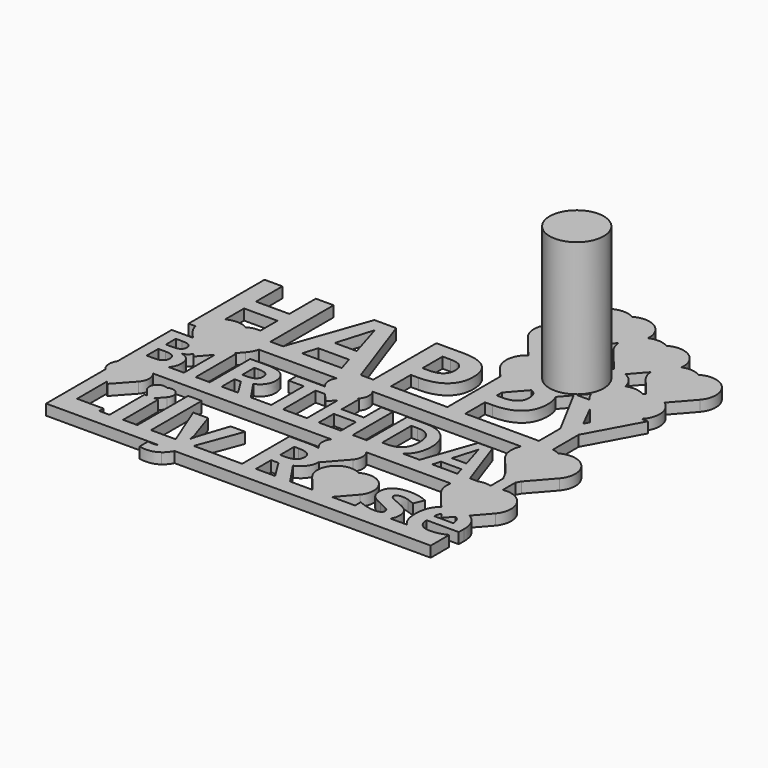
from build123d import *

# Parameters (mm, degrees)
F0_TEXT_SIZE   = 22.0588235294
F0_TEXT_SIZE_2 = 14.6296860713
F0_W           = 2.5421468203
F0_H           = 9.3203158344
F0_H_2         = 12.9721510883
F1_DEPTH       = 2
F2_W           = 69.2715635477
F2_H           = 3
F2_W_2         = 71.8336534358
F2_W_3         = 66.3625919118
F3_DEPTH       = 2
F5_DEPTH       = 2
F6_R           = 5.0531833036
F7_DEPTH       = 25


# Not quite as in the source:
# - Text() gives the source's letters only with a copy of the font that has no kerning and outlines rounded to 1/6400 em; it was checked with that copy


with BuildPart() as f1:
    # F0 (on Top) → F1 (new body)
    with BuildSketch(Plane.XY):
        with Locations((-37.5, 11.5387746485)):
            Text('HAPPY', F0_TEXT_SIZE, font='Open Sans', font_style=FontStyle.BOLD, text_align=(TextAlign.LEFT, TextAlign.BOTTOM))
        with Locations((-37.5, -3.9945993228)):
            Text('BIRTHDAY', F0_TEXT_SIZE_2, font='Open Sans', font_style=FontStyle.BOLD, text_align=(TextAlign.LEFT, TextAlign.BOTTOM))
        Polygon((-35.9661758429, -9.0986326135), (-35.9661758429, -21.2865327415), (-28.4384336321, -21.2865327415), (-28.4384336321, -19.152516523), (-33.3813486983, -19.152516523), (-33.3813486983, -9.0986326135), align=None)
        with Locations((-25.2494131455, -16.6263748243)):
            Rectangle(F0_W, F0_H)
        with Locations((-20.0397460521, -14.8004571973)):
            Rectangle(F0_W, F0_H_2)
        with BuildLine():
            Line((-14.6500213402, -11.9662169071), (-17.4349125053, -11.9662169071))
            Line((-17.4349125053, -11.9662169071), (-13.7323943662, -21.2198447347))
            Line((-13.7323943662, -21.2198447347), (-13.8844430218, -21.6786582217))
            add(Edge.make_bspline(
                [(-14.6713615023, -22.9243901892), (-14.1672001707, -22.5109245469), (-13.8844430218, -21.6786582217)],
                knots=[0, 0, 0, 1, 1, 1], degree=2))
            add(Edge.make_bspline(
                [(-15.8504054631, -23.3378558316), (-15.175522834, -23.3378558316), (-14.6713615023, -22.9243901892)],
                knots=[0, 0, 0, 1, 1, 1], degree=2))
            add(Edge.make_bspline(
                [(-16.8507255655, -23.2284875004), (-16.3919120785, -23.3378558316), (-15.8504054631, -23.3378558316)],
                knots=[0, 0, 0, 1, 1, 1], degree=2))
            Line((-16.8507255655, -23.2284875004), (-16.8507255655, -25.2451328269))
            add(Edge.make_bspline(
                [(-15.5596457533, -25.3891789216), (-16.2185232608, -25.3891789216), (-16.8507255655, -25.2451328269)],
                knots=[0, 0, 0, 1, 1, 1], degree=2))
            add(Edge.make_bspline(
                [(-13.2135616731, -24.6636134073), (-14.2178830559, -25.3891789216), (-15.5596457533, -25.3891789216)],
                knots=[0, 0, 0, 1, 1, 1], degree=2))
            add(Edge.make_bspline(
                [(-11.6650661545, -22.4789143036), (-12.2092402902, -23.938047893), (-13.2135616731, -24.6636134073)],
                knots=[0, 0, 0, 1, 1, 1], degree=2))
            Line((-11.6650661545, -22.4789143036), (-7.7224711908, -11.9662169071))
            Line((-7.7224711908, -11.9662169071), (-10.4486769099, -11.9662169071))
            Line((-10.4486769099, -11.9662169071), (-12.1745625267, -17.2105617641))
            add(Edge.make_bspline(
                [(-12.5320102433, -18.8270790497), (-12.441314554, -17.9681375217), (-12.1745625267, -17.2105617641)],
                knots=[0, 0, 0, 1, 1, 1], degree=2))
            Line((-12.5320102433, -18.8270790497), (-12.5826931285, -18.8270790497))
            add(Edge.make_bspline(
                [(-12.8921254802, -17.2105617641), (-12.6653862569, -17.8934469541), (-12.5826931285, -18.8270790497)],
                knots=[0, 0, 0, 1, 1, 1], degree=2))
            Line((-12.8921254802, -17.2105617641), (-14.6500213402, -11.9662169071))
        make_face()
        with BuildLine():
            Line((0.8322663252, -21.2865327415), (0.8322663252, -16.6103697027))
            Line((0.8322663252, -16.6103697027), (2.2060392659, -16.6103697027))
            Line((2.2060392659, -16.6103697027), (5.1163038839, -21.2865327415))
            Line((5.1163038839, -21.2865327415), (7.9838881776, -21.2865327415))
            add(Edge.make_bspline(
                [(4.3987409304, -15.9754998777), (7.1516218523, -20.0861486186), (7.9838881776, -21.2865327415)],
                knots=[0, 0, 0, 1, 1, 1], degree=2))
            add(Edge.make_bspline(
                [(6.0752774221, -14.6630799033), (5.4844216816, -15.5006812691), (4.3987409304, -15.9754998777)],
                knots=[0, 0, 0, 1, 1, 1], degree=2))
            add(Edge.make_bspline(
                [(6.6661331626, -12.7504678674), (6.6661331626, -13.8254785375), (6.0752774221, -14.6630799033)],
                knots=[0, 0, 0, 1, 1, 1], degree=2))
            add(Edge.make_bspline(
                [(5.4750853606, -10.0029219861), (6.6661331626, -10.9072113587), (6.6661331626, -12.7504678674)],
                knots=[0, 0, 0, 1, 1, 1], degree=2))
            add(Edge.make_bspline(
                [(1.7979086641, -9.0986326135), (4.2840375587, -9.0986326135), (5.4750853606, -10.0029219861)],
                knots=[0, 0, 0, 1, 1, 1], degree=2))
            Line((1.7979086641, -9.0986326135), (-1.7525608195, -9.0986326135))
            Line((-1.7525608195, -9.0986326135), (-1.7525608195, -21.2865327415))
            Line((-1.7525608195, -21.2865327415), (0.8322663252, -21.2865327415))
        make_face()
        with BuildLine():
            Line((1.6645326504, -14.5083637274), (0.8322663252, -14.5083637274))
            Line((0.8322663252, -14.5083637274), (0.8322663252, -11.2166437104))
            Line((0.8322663252, -11.2166437104), (1.6165172855, -11.2166437104))
            add(Edge.make_bspline(
                [(3.4611075544, -11.5834277479), (2.8649167734, -11.2166437104), (1.6165172855, -11.2166437104)],
                knots=[0, 0, 0, 1, 1, 1], degree=2))
            add(Edge.make_bspline(
                [(4.0572983355, -12.8171558743), (4.0572983355, -11.9502117855), (3.4611075544, -11.5834277479)],
                knots=[0, 0, 0, 1, 1, 1], degree=2))
            add(Edge.make_bspline(
                [(3.4744451558, -14.1002331256), (4.0572983355, -13.6921025239), (4.0572983355, -12.8171558743)],
                knots=[0, 0, 0, 1, 1, 1], degree=2))
            add(Edge.make_bspline(
                [(1.6645326504, -14.5083637274), (2.8915919761, -14.5083637274), (3.4744451558, -14.1002331256)],
                knots=[0, 0, 0, 1, 1, 1], degree=2))
        make_face(mode=Mode.SUBTRACT)
        with BuildLine():
            add(Edge.make_bspline(
                [(26.3924455826, -18.517646698), (26.3924455826, -19.9527726049), (25.3961267606, -20.7036795618)],
                knots=[0, 0, 0, 1, 1, 1], degree=2))
            add(Edge.make_bspline(
                [(26.1497012377, -17.326598896), (26.3924455826, -17.8267589472), (26.3924455826, -18.517646698)],
                knots=[0, 0, 0, 1, 1, 1], degree=2))
            add(Edge.make_bspline(
                [(25.3987942808, -16.4436496856), (25.9069568929, -16.8264388448), (26.1497012377, -17.326598896)],
                knots=[0, 0, 0, 1, 1, 1], degree=2))
            add(Edge.make_bspline(
                [(23.7996158771, -15.6180521611), (24.8906316688, -16.0608605264), (25.3987942808, -16.4436496856)],
                knots=[0, 0, 0, 1, 1, 1], degree=2))
            add(Edge.make_bspline(
                [(22.2097737943, -14.8764815251), (22.5725565514, -15.1272284308), (23.7996158771, -15.6180521611)],
                knots=[0, 0, 0, 1, 1, 1], degree=2))
            add(Edge.make_bspline(
                [(21.8469910371, -14.2842920245), (21.8469910371, -14.6257346195), (22.2097737943, -14.8764815251)],
                knots=[0, 0, 0, 1, 1, 1], degree=2))
            add(Edge.make_bspline(
                [(22.9726845924, -13.6760974022), (21.8469910371, -13.6760974022), (21.8469910371, -14.2842920245)],
                knots=[0, 0, 0, 1, 1, 1], degree=2))
            add(Edge.make_bspline(
                [(24.2157490397, -13.8681588619), (23.6075544174, -13.6760974022), (22.9726845924, -13.6760974022)],
                knots=[0, 0, 0, 1, 1, 1], degree=2))
            add(Edge.make_bspline(
                [(25.5255014938, -14.3589825921), (24.823943662, -14.0602203215), (24.2157490397, -13.8681588619)],
                knots=[0, 0, 0, 1, 1, 1], degree=2))
            Line((25.5255014938, -14.3589825921), (26.2910798122, -12.5263961645))
            add(Edge.make_bspline(
                [(23.0153649168, -11.7928280894), (24.6985702091, -11.7928280894), (26.2910798122, -12.5263961645)],
                knots=[0, 0, 0, 1, 1, 1], degree=2))
            add(Edge.make_bspline(
                [(20.2851579172, -12.4717119989), (21.2467989757, -11.7928280894), (23.0153649168, -11.7928280894)],
                knots=[0, 0, 0, 1, 1, 1], degree=2))
            add(Edge.make_bspline(
                [(19.3235168587, -14.3936603557), (19.3235168587, -13.1505959084), (20.2851579172, -12.4717119989)],
                knots=[0, 0, 0, 1, 1, 1], degree=2))
            add(Edge.make_bspline(
                [(19.5515898421, -15.6127171205), (19.3235168587, -15.1165583497), (19.3235168587, -14.3936603557)],
                knots=[0, 0, 0, 1, 1, 1], degree=2))
            add(Edge.make_bspline(
                [(20.2851579172, -16.4929988107), (19.7796628254, -16.1088758913), (19.5515898421, -15.6127171205)],
                knots=[0, 0, 0, 1, 1, 1], degree=2))
            add(Edge.make_bspline(
                [(21.865663679, -17.3279326562), (20.790653009, -16.87712173), (20.2851579172, -16.4929988107)],
                knots=[0, 0, 0, 1, 1, 1], degree=2))
            add(Edge.make_bspline(
                [(23.0647140418, -17.8801093527), (22.6152368758, -17.6427000484), (21.865663679, -17.3279326562)],
                knots=[0, 0, 0, 1, 1, 1], degree=2))
            add(Edge.make_bspline(
                [(23.6982501067, -18.3055788363), (23.5141912079, -18.117518657), (23.0647140418, -17.8801093527)],
                knots=[0, 0, 0, 1, 1, 1], degree=2))
            add(Edge.make_bspline(
                [(23.8823090055, -18.7950688064), (23.8823090055, -18.4936390155), (23.6982501067, -18.3055788363)],
                knots=[0, 0, 0, 1, 1, 1], degree=2))
            add(Edge.make_bspline(
                [(22.4978659838, -19.5953248883), (23.8823090055, -19.5953248883), (23.8823090055, -18.7950688064)],
                knots=[0, 0, 0, 1, 1, 1], degree=2))
            add(Edge.make_bspline(
                [(20.9346991037, -19.3699194253), (21.8229833547, -19.5953248883), (22.4978659838, -19.5953248883)],
                knots=[0, 0, 0, 1, 1, 1], degree=2))
            add(Edge.make_bspline(
                [(19.3395219804, -18.811073928), (20.0464148528, -19.1445139622), (20.9346991037, -19.3699194253)],
                knots=[0, 0, 0, 1, 1, 1], degree=2))
            Line((19.3395219804, -18.811073928), (19.3395219804, -20.910412383))
            add(Edge.make_bspline(
                [(20.6812846778, -21.3158754645), (19.9637217243, -21.1771644103), (19.3395219804, -20.910412383)],
                knots=[0, 0, 0, 1, 1, 1], degree=2))
            add(Edge.make_bspline(
                [(22.4151728553, -21.4545865187), (21.3988476312, -21.4545865187), (20.6812846778, -21.3158754645)],
                knots=[0, 0, 0, 1, 1, 1], degree=2))
            add(Edge.make_bspline(
                [(25.3961267606, -20.7036795618), (24.3998079385, -21.4545865187), (22.4151728553, -21.4545865187)],
                knots=[0, 0, 0, 1, 1, 1], degree=2))
        make_face()
        with BuildLine():
            add(Edge.make_bspline(
                [(32.5917626974, -21.4545865187), (30.3430431071, -21.4545865187), (29.0759709774, -20.2115220714)],
                knots=[0, 0, 0, 1, 1, 1], degree=2))
            add(Edge.make_bspline(
                [(34.443021767, -21.2918677821), (33.6854460094, -21.4545865187), (32.5917626974, -21.4545865187)],
                knots=[0, 0, 0, 1, 1, 1], degree=2))
            add(Edge.make_bspline(
                [(35.8674775928, -20.7957090113), (35.2005975245, -21.1291490454), (34.443021767, -21.2918677821)],
                knots=[0, 0, 0, 1, 1, 1], degree=2))
            Line((35.8674775928, -20.7957090113), (35.8674775928, -18.8270790497))
            add(Edge.make_bspline(
                [(34.3016431925, -19.3859245469), (35.0512163892, -19.211201969), (35.8674775928, -18.8270790497)],
                knots=[0, 0, 0, 1, 1, 1], degree=2))
            add(Edge.make_bspline(
                [(32.7091335894, -19.5606471248), (33.5520699957, -19.5606471248), (34.3016431925, -19.3859245469)],
                knots=[0, 0, 0, 1, 1, 1], degree=2))
            add(Edge.make_bspline(
                [(31.0259282971, -18.9524525025), (31.6261203585, -19.5606471248), (32.7091335894, -19.5606471248)],
                knots=[0, 0, 0, 1, 1, 1], degree=2))
            add(Edge.make_bspline(
                [(30.3830559112, -17.2612446493), (30.4257362356, -18.3442578802), (31.0259282971, -18.9524525025)],
                knots=[0, 0, 0, 1, 1, 1], degree=2))
            Line((30.3830559112, -17.2612446493), (36.3929790866, -17.2612446493))
            Line((36.3929790866, -17.2612446493), (36.3929790866, -16.0261827629))
            add(Edge.make_bspline(
                [(35.292626974, -12.9171878845), (36.3929790866, -14.0415476796), (36.3929790866, -16.0261827629)],
                knots=[0, 0, 0, 1, 1, 1], degree=2))
            add(Edge.make_bspline(
                [(32.2183098592, -11.7928280894), (34.1922748613, -11.7928280894), (35.292626974, -12.9171878845)],
                knots=[0, 0, 0, 1, 1, 1], degree=2))
            add(Edge.make_bspline(
                [(28.9799402475, -13.0719040603), (30.1509816475, -11.7928280894), (32.2183098592, -11.7928280894)],
                knots=[0, 0, 0, 1, 1, 1], degree=2))
            add(Edge.make_bspline(
                [(27.8088988476, -16.6930628312), (27.8088988476, -14.3509800313), (28.9799402475, -13.0719040603)],
                knots=[0, 0, 0, 1, 1, 1], degree=2))
            add(Edge.make_bspline(
                [(29.0759709774, -20.2115220714), (27.8088988476, -18.9684576242), (27.8088988476, -16.6930628312)],
                knots=[0, 0, 0, 1, 1, 1], degree=2))
        make_face()
        with BuildLine():
            add(Edge.make_bspline(
                [(32.2343149808, -13.6014068346), (31.426056338, -13.6014068346), (30.967242851, -14.113570727)],
                knots=[0, 0, 0, 1, 1, 1], degree=2))
            add(Edge.make_bspline(
                [(33.5173922322, -14.113570727), (33.0425736236, -13.6014068346), (32.2343149808, -13.6014068346)],
                knots=[0, 0, 0, 1, 1, 1], degree=2))
            add(Edge.make_bspline(
                [(34.0108834827, -15.5673692759), (33.9922108408, -14.6257346195), (33.5173922322, -14.113570727)],
                knots=[0, 0, 0, 1, 1, 1], degree=2))
            Line((34.0108834827, -15.5673692759), (30.4417413572, -15.5673692759))
            add(Edge.make_bspline(
                [(30.967242851, -14.113570727), (30.5084293641, -14.6257346195), (30.4417413572, -15.5673692759)],
                knots=[0, 0, 0, 1, 1, 1], degree=2))
        make_face(mode=Mode.SUBTRACT)
    extrude(amount=F1_DEPTH)

    # F2 (on Top) → F3 (join)
    with BuildSketch(Plane.XY):
        with Locations((-1.5498323682, -4.4945993228)):
            Rectangle(F2_W, F2_H)
        with Locations((-0.0493491251, -21.652516523)):
            Rectangle(F2_W_2, F2_H)
        with Locations((-2.3368566176, 11.0387746485)):
            Rectangle(F2_W_3, F2_H)
    extrude(amount=F3_DEPTH)

    # F4 (on Top) → F5 (join)
    with BuildSketch(Plane.XY):
        with BuildLine():
            ThreePointArc((15.8710453597, 42.3152042751), (13.5240060481, 43.5901863002), (10.8977104083, 43.1036229369))
            ThreePointArc((10.8977104083, 43.1036229369), (10.6969632271, 43.2120119507), (10.4903631205, 43.3087797398))
            Line((10.4903631205, 43.3087797398), (13.5120771973, 39.6303699124))
            Line((13.5120771973, 39.6303699124), (15.8710453597, 42.3152042751))
        make_face()
        with BuildLine():
            ThreePointArc((10.4903631205, 43.3087797398), (10.6969632271, 43.2120119507), (10.8977104083, 43.1036229369))
            ThreePointArc((10.8977104083, 43.1036229369), (13.5240060481, 43.5901863002), (15.8710453597, 42.3152042751))
            Line((15.8710453597, 42.3152042751), (17.28911835, 43.9291688694))
            ThreePointArc((17.28911835, 43.9291688694), (17.8752784968, 46.2349552383), (19.667146129, 47.8000254877))
            ThreePointArc((19.667146129, 47.8000254877), (17.8364951333, 51.5292442561), (13.6832215476, 51.6223797092))
            ThreePointArc((13.6832215476, 51.6223797092), (8.632499056, 50.7453792284), (8.5923837689, 45.6192385462))
            Line((8.5923837689, 45.6192385462), (10.4903631205, 43.3087797398))
        make_face()
        with BuildLine():
            Line((13.5120771973, 39.6303699124), (10.4903631205, 43.3087797398))
            ThreePointArc((10.4903631205, 43.3087797398), (5.7044549328, 42.0484877948), (5.8068726296, 37.1004817739))
            Line((5.8068726296, 37.1004817739), (9.434985023, 32.6838877668))
            ThreePointArc((9.434985023, 32.6838877668), (11.0020288677, 33.3963663052), (12.7233963769, 33.3842841927))
            Line((12.7233963769, 33.3842841927), (15.988548187, 37.1004817739))
            ThreePointArc((15.988548187, 37.1004817739), (16.8966953315, 39.7296300543), (15.8710453597, 42.3152042751))
            Line((15.8710453597, 42.3152042751), (13.5120771973, 39.6303699124))
        make_face()
        with BuildLine():
            Line((18.7740593263, 45.6192385462), (17.28911835, 43.9291688694))
            ThreePointArc((17.28911835, 43.9291688694), (17.5547067733, 42.6933470485), (18.1926598963, 41.6021052805))
            Line((18.1926598963, 41.6021052805), (21.9117701176, 37.0747372903))
            ThreePointArc((21.9117701176, 37.0747372903), (23.0705080697, 37.1278805872), (24.1957729049, 36.8463190445))
            Line((24.1957729049, 36.8463190445), (26.6866230167, 39.6812534361))
            ThreePointArc((26.6866230167, 39.6812534361), (27.3192394754, 42.0896780932), (29.2541092545, 43.6571575508))
            ThreePointArc((29.2541092545, 43.6571575508), (27.4897793831, 47.4776581319), (23.2834976751, 47.6052464435))
            ThreePointArc((23.2834976751, 47.6052464435), (21.4986284564, 48.1353554822), (19.667146129, 47.8000254877))
            ThreePointArc((19.667146129, 47.8000254877), (19.3848459929, 46.6423702915), (18.7740593263, 45.6192385462))
        make_face()
        with BuildLine():
            ThreePointArc((19.667146129, 47.8000254877), (17.8752784968, 46.2349552383), (17.28911835, 43.9291688694))
            Line((17.28911835, 43.9291688694), (18.7740593263, 45.6192385462))
            ThreePointArc((18.7740593263, 45.6192385462), (19.3848459929, 46.6423702915), (19.667146129, 47.8000254877))
        make_face()
        with BuildLine():
            ThreePointArc((12.7233963769, 33.3842841927), (11.0020288677, 33.3963663052), (9.434985023, 32.6838877668))
            Line((9.434985023, 32.6838877668), (10.726566058, 31.1116131401))
            Line((10.726566058, 31.1116131401), (12.7233963769, 33.3842841927))
        make_face()
        with BuildLine():
            Line((10.726566058, 31.1116131401), (9.434985023, 32.6838877668))
            ThreePointArc((9.434985023, 32.6838877668), (7.8639413359, 29.961977531), (8.7444575695, 26.9450809863))
            Line((8.7444575695, 26.9450809863), (13.6641509979, 20.9562123525))
            Line((13.6641509979, 20.9562123525), (18.7530286138, 26.7480639377))
            Line((18.7530286138, 26.7480639377), (15.5816244153, 30.6086953786))
            ThreePointArc((15.5816244153, 30.6086953786), (14.8796431709, 31.877095773), (14.6758527891, 33.3123959883))
            ThreePointArc((14.6758527891, 33.3123959883), (14.2451145511, 33.1544509053), (13.8352953482, 32.9482221494))
            ThreePointArc((13.8352953482, 32.9482221494), (13.2957128961, 33.2079868833), (12.7233963769, 33.3842841927))
            Line((12.7233963769, 33.3842841927), (10.726566058, 31.1116131401))
        make_face()
        with BuildLine():
            Line((23.1123533248, 35.6132366467), (21.9117701176, 37.0747372903))
            ThreePointArc((21.9117701176, 37.0747372903), (21.2728463678, 36.8948772429), (20.672462194, 36.6118365416))
            ThreePointArc((20.672462194, 36.6118365416), (16.7442015088, 36.6522763701), (14.6758527891, 33.3123959883))
            ThreePointArc((14.6758527891, 33.3123959883), (19.1621928454, 31.7048755956), (18.9261331269, 26.9450809863))
            Line((18.9261331269, 26.9450809863), (18.7530286138, 26.7480639377))
            Line((18.7530286138, 26.7480639377), (20.5013178437, 24.6198267448))
            Line((20.5013178437, 24.6198267448), (24.2263502902, 28.8594325496))
            ThreePointArc((24.2263502902, 28.8594325496), (24.4135741152, 31.8368320124), (26.6091530057, 33.8565829024))
            ThreePointArc((26.6091530057, 33.8565829024), (25.7849426689, 35.6601969249), (24.1957729049, 36.8463190445))
            Line((24.1957729049, 36.8463190445), (23.1123533248, 35.6132366467))
        make_face()
        with BuildLine():
            ThreePointArc((18.9261331269, 26.9450809863), (19.1621928454, 31.7048755956), (14.6758527891, 33.3123959883))
            ThreePointArc((14.6758527891, 33.3123959883), (14.8796431709, 31.877095773), (15.5816244153, 30.6086953786))
            Line((15.5816244153, 30.6086953786), (18.7530286138, 26.7480639377))
            Line((18.7530286138, 26.7480639377), (18.9261331269, 26.9450809863))
        make_face()
        with BuildLine():
            ThreePointArc((28.3743354538, 41.6021052805), (28.9607013297, 42.566923344), (29.2541092545, 43.6571575508))
            ThreePointArc((29.2541092545, 43.6571575508), (27.3192394754, 42.0896780932), (26.6866230167, 39.6812534361))
            Line((26.6866230167, 39.6812534361), (28.3743354538, 41.6021052805))
        make_face()
        with BuildLine():
            ThreePointArc((32.6795068222, 43.3838480601), (30.9976522422, 43.9070743086), (29.2541092545, 43.6571575508))
            ThreePointArc((29.2541092545, 43.6571575508), (28.9607013297, 42.566923344), (28.3743354538, 41.6021052805))
            Line((28.3743354538, 41.6021052805), (26.6866230167, 39.6812534361))
            ThreePointArc((26.6866230167, 39.6812534361), (26.9555430113, 38.4595774361), (27.5886690435, 37.3807068971))
            Line((27.5886690435, 37.3807068971), (30.5142626527, 33.8193069732))
            ThreePointArc((30.5142626527, 33.8193069732), (32.4509480968, 34.0923705397), (34.2855856515, 33.414565801))
            Line((34.2855856515, 33.414565801), (37.7703446009, 37.3807068971))
            ThreePointArc((37.7703446009, 37.3807068971), (37.7302293138, 42.5068475793), (32.6795068222, 43.3838480601))
        make_face()
        with BuildLine():
            ThreePointArc((30.0241161722, 33.5793105403), (28.347824397, 34.1020890319), (26.6091530057, 33.8565829024))
            ThreePointArc((26.6091530057, 33.8565829024), (26.5433448923, 32.1396341697), (25.7632999727, 30.6086953786))
            Line((25.7632999727, 30.6086953786), (24.2263502902, 28.8594325496))
            ThreePointArc((24.2263502902, 28.8594325496), (24.5205599516, 28.1851587162), (24.9332783935, 27.5761693773))
            Line((24.9332783935, 27.5761693773), (29.8529718219, 21.5873007435))
            Line((29.8529718219, 21.5873007435), (34.9397683559, 27.3767837676))
            ThreePointArc((34.9397683559, 27.3767837676), (36.0008422313, 30.5460799625), (34.2855856515, 33.414565801))
            Line((34.2855856515, 33.414565801), (32.508362472, 31.3918382633))
            Line((32.508362472, 31.3918382633), (30.5142626527, 33.8193069732))
            ThreePointArc((30.5142626527, 33.8193069732), (30.2650915834, 33.7076777832), (30.0241161722, 33.5793105403))
        make_face()
        with BuildLine():
            ThreePointArc((25.7632999727, 30.6086953786), (26.5433448923, 32.1396341697), (26.6091530057, 33.8565829024))
            ThreePointArc((26.6091530057, 33.8565829024), (24.4135741152, 31.8368320124), (24.2263502902, 28.8594325496))
            Line((24.2263502902, 28.8594325496), (25.7632999727, 30.6086953786))
        make_face()
        with BuildLine():
            Line((32.508362472, 31.3918382633), (34.2855856515, 33.414565801))
            ThreePointArc((34.2855856515, 33.414565801), (32.4509480968, 34.0923705397), (30.5142626527, 33.8193069732))
            Line((30.5142626527, 33.8193069732), (32.508362472, 31.3918382633))
        make_face()
        with BuildLine():
            ThreePointArc((-23.460767245, -10.5974629963), (-23.3785588051, -8.6388796142), (-25.3041368139, -8.2715154565))
            ThreePointArc((-25.3041368139, -8.2715154565), (-27.1981577482, -8.6003906368), (-27.2132009809, -10.5226933926))
            Line((-27.2132009809, -10.5226933926), (-25.3683159452, -12.7685191303))
            Line((-25.3683159452, -12.7685191303), (-23.460767245, -10.5974629963))
        make_face()
        with BuildLine():
            ThreePointArc((17.7506930834, -17.0362158441), (17.7155922072, -12.5508427471), (13.296210027, -11.7834673264))
            ThreePointArc((13.296210027, -11.7834673264), (8.8768278469, -12.5508427471), (8.8417269707, -17.0362158441))
            Line((8.8417269707, -17.0362158441), (13.1464587205, -22.2764758987))
            Line((13.1464587205, -22.2764758987), (17.7506930834, -17.0362158441))
        make_face()
        with BuildLine():
            ThreePointArc((37.2771124401, 5.1807187554), (37.236997153, 10.3068594377), (32.1862746614, 11.1838599185))
            ThreePointArc((32.1862746614, 11.1838599185), (27.1355521698, 10.3068594377), (27.0954368827, 5.1807187554))
            Line((27.0954368827, 5.1807187554), (32.0151303111, -0.8081498784))
            Line((32.0151303111, -0.8081498784), (37.2771124401, 5.1807187554))
        make_face()
        with BuildLine():
            ThreePointArc((-23.3789527746, 7.6379913258), (-23.1597302683, 12.8608803447), (-28.2946049583, 13.8405180985))
            ThreePointArc((-28.2946049583, 13.8405180985), (-33.3453274499, 12.9635176177), (-33.385442737, 7.8373769355))
            Line((-33.385442737, 7.8373769355), (-28.4657493086, 1.8485083017))
            Line((-28.4657493086, 1.8485083017), (-23.3789527746, 7.6379913258))
        make_face()
        with BuildLine():
            ThreePointArc((36.8976171174, -9.3308138604), (36.8575018303, -4.2046731782), (31.8067793387, -3.3276726974))
            ThreePointArc((31.8067793387, -3.3276726974), (26.7560568471, -4.2046731782), (26.71594156, -9.3308138604))
            Line((26.71594156, -9.3308138604), (31.6356349884, -15.3196824942))
            Line((31.6356349884, -15.3196824942), (36.8976171174, -9.3308138604))
        make_face()
        with BuildLine():
            ThreePointArc((-29.7967798697, -9.3315176463), (-29.6597658033, -6.0672120096), (-32.8690624845, -5.4549384134))
            ThreePointArc((-32.8690624845, -5.4549384134), (-36.0630556223, -6.0480952208), (-35.9745223626, -9.2954924901))
            Line((-35.9745223626, -9.2954924901), (-32.8690624845, -12.7345188382))
            Line((-32.8690624845, -12.7345188382), (-29.7967798697, -9.3315176463))
        make_face()
        with BuildLine():
            ThreePointArc((-1.4179188738, 6.4611722219), (-1.2809048074, 9.7254778587), (-4.4902014886, 10.3377514548))
            ThreePointArc((-4.4902014886, 10.3377514548), (-7.6469030459, 9.7896261543), (-7.6719751003, 6.5857882279))
            Line((-7.6719751003, 6.5857882279), (-4.5971667076, 2.8427453318))
            Line((-4.5971667076, 2.8427453318), (-1.4179188738, 6.4611722219))
        make_face()
        with BuildLine():
            ThreePointArc((10.0142014591, -9.0243846608), (9.9891294046, -5.8205467344), (6.8324278474, -5.2724214339))
            ThreePointArc((6.8324278474, -5.2724214339), (3.6757262901, -5.8205467344), (3.6506542357, -9.0243846608))
            Line((3.6506542357, -9.0243846608), (6.7254626285, -12.7674275569))
            Line((6.7254626285, -12.7674275569), (10.0142014591, -9.0243846608))
        make_face()
        with BuildLine():
            ThreePointArc((24.1957729049, 36.8463190445), (23.0705080697, 37.1278805872), (21.9117701176, 37.0747372903))
            Line((21.9117701176, 37.0747372903), (23.1123533248, 35.6132366467))
            Line((23.1123533248, 35.6132366467), (24.1957729049, 36.8463190445))
        make_face()
    extrude(amount=F5_DEPTH)

    # F6 (on face) → F7 (join)
    with BuildSketch(Plane.XY.offset(2)):
        with Locations((19.4810219109, 31.4199179411)):
            Circle(F6_R)
    extrude(amount=F7_DEPTH)


solid = f1.part
